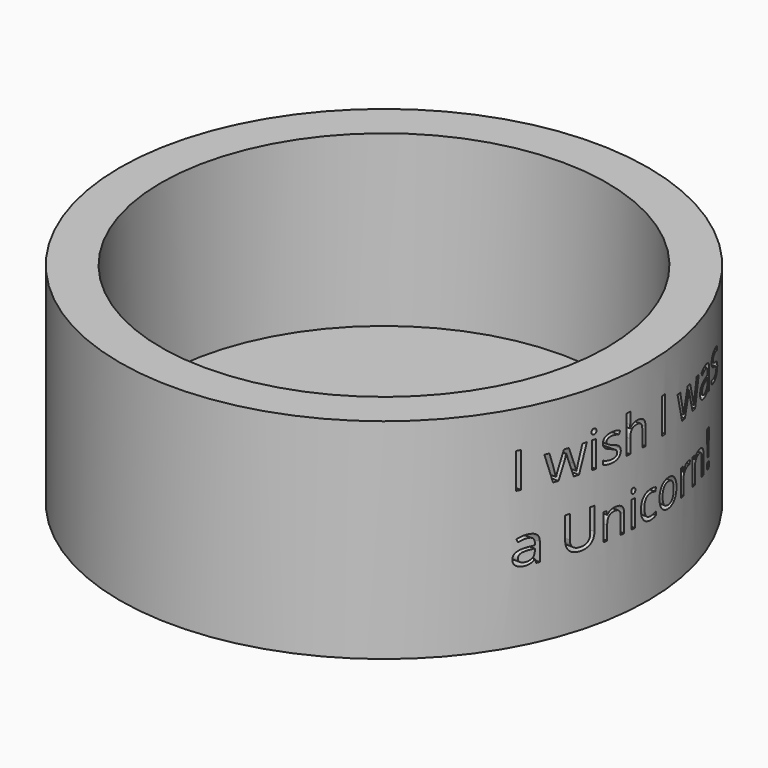
from build123d import *

# Parameters (mm, degrees)
F3_TEXT_SIZE = 10.5833333333
F4_DEPTH     = 114.3


# Not quite as in the source:
# - Text() gives the source's letters only with a copy of the font that has no kerning and outlines rounded to 1/6400 em; it was checked with that copy


with BuildPart() as f1:
    # F0 (on Front) → F1 (revolve)
    with BuildSketch(Plane.XZ):
        Polygon((8.8322721422, 44.8887273669), (0, 44.8887273669), (0, 0), (56.6304549575, 0), (56.6304549575, 8.5205454379), (8.8322721422, 8.5205454379), align=None)
    revolve(axis=Axis((56.6304549575, 0, 4.260272719), (0, 0, -1)))

    # F3 (on offset) → F4 (cut)
    with BuildSketch(Plane.YZ.offset(57.15)):
        with Locations((-27.9846484375, 29.3976113178)):
            Text('I wish I was', F3_TEXT_SIZE, font='Open Sans', text_align=(TextAlign.LEFT, TextAlign.BOTTOM))
        with Locations((-27.9846484375, 15.0042779845)):
            Text('a Unicorn!', F3_TEXT_SIZE, font='Open Sans', text_align=(TextAlign.LEFT, TextAlign.BOTTOM))
    extrude(amount=F4_DEPTH, mode=Mode.SUBTRACT)


solid = f1.part
